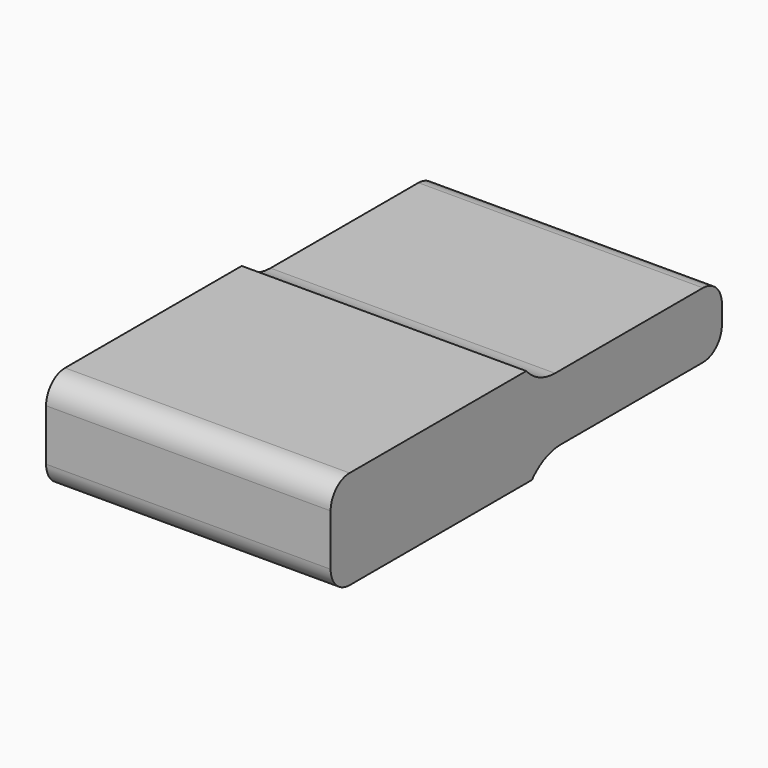
from build123d import *

# Parameters (mm, degrees)
F0_W        = 30.5091738701
F0_H        = 52.441470325
F1_DEPTH    = 10.5918
F3_DEPTH    = 1.778
F5_DEPTH    = 1.778
F6_T1_DEPTH = 30.5091738701
F6_T6_DEPTH = 49.8209621392
F7_R        = 2.54


# Not quite as in the source:
# - a fillet or chamfer that OpenCascade refuses, or shapes differently, is made with other operations: its cross-section is extruded or revolved along the edge and cut away or added


with BuildPart() as f1:
    # F0 (on Top) → F1 (new body)
    with BuildSketch(Plane.XY):
        with Locations((15.254586935, 26.2207351625)):
            Rectangle(F0_W, F0_H)
    extrude(amount=F1_DEPTH)

    # F2 (on face) → F3 (cut)
    with BuildSketch(Plane.XY.offset(10.5918)):
        Polygon((27.9714719847, 52.441470325), (0, 52.441470325), (0, 27.7975574136), (0, 26.2207351625), (30.5091738701, 26.2207351625), (30.5091738701, 52.4368782499), align=None)
    extrude(amount=-F3_DEPTH, mode=Mode.SUBTRACT)

    # F4 (on face) → F5 (cut)
    with BuildSketch(Plane(origin=(0, 0, 0), x_dir=(1, 0, 0), z_dir=(0, 0, -1))):
        Polygon((30.5091738701, -26.980528608), (0, -26.2207351625), (0, -52.441470325), (30.5091738701, -52.441470325), align=None)
    extrude(amount=-F5_DEPTH, mode=Mode.SUBTRACT)

    # F6: fillet of radius 5.08 on 2 edges, made by hand

    # F6_s2 → F6_t1 (join)
    with BuildSketch(Plane.YZ):
        with BuildLine():
            ThreePointArc((26.2207351625, 10.5918), (27.9560844701, 9.2796608604), (30.0812009375, 8.8138))
            Line((30.0812009375, 8.8138), (26.2207351625, 8.8138))
            Line((26.2207351625, 8.8138), (26.2207351625, 10.5918))
        make_face()
    extrude(amount=F6_T1_DEPTH)


with BuildPart() as f6_tool4:
    # F6_s5 → F6_t6 (new body)
    with BuildSketch(Plane(origin=(40.8099373033, 1.0163212877, 0), x_dir=(0, 0, 1), z_dir=(-0.9996900453, -0.0248960508, 0))):
        with BuildLine():
            ThreePointArc((1.778, 30.0730736971), (1.3121391396, 27.9479572297), (0, 26.2126079221))
            Line((0, 26.2126079221), (1.778, 26.2126079221))
            Line((1.778, 26.2126079221), (1.778, 30.0730736971))
        make_face()
    extrude(amount=F6_T6_DEPTH)

    split(bisect_by=Plane.YZ, keep=Keep.TOP)

    split(bisect_by=Plane.YZ.offset(30.5091738701), keep=Keep.BOTTOM)


with BuildPart() as f1_1:
    add(f1.part)

    # F6_t3: union F6_tool4
    add(f6_tool4.part)

    # F7
    f7_edges = [f1_1.edges().sort_by_distance(p)[0] for p in [
        (15.254587, 52.44147, 1.778),
        (15.254587, 0, 0),
        (15.254587, 0, 10.5918),
        (13.985736, 52.44147, 8.8138),
    ]]
    fillet(f7_edges, radius=F7_R)


solid = f1_1.part
